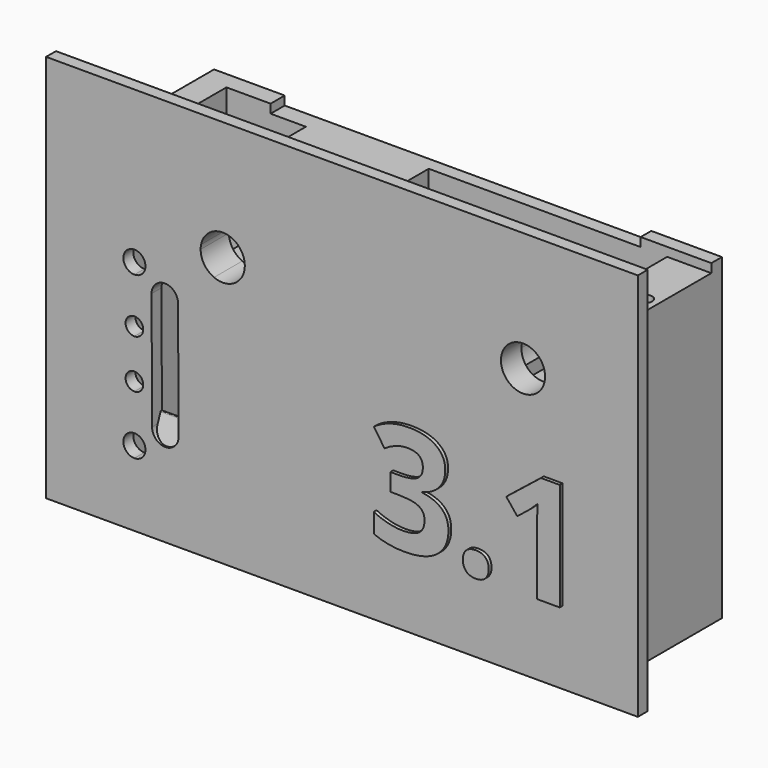
from build123d import *

# Parameters (mm, degrees)
F1_DEPTH      = 15
F2_W          = 15
F2_H          = 4
F3_DEPTH      = 25
F3_DEPTH_BACK = 1
F6_DEPTH      = 25
F7_DEPTH      = 15
F9_DEPTH      = 25
F10_W         = 27
F10_H         = 15
F11_DEPTH     = 2
F12_W         = 48
F12_H         = 36
F13_DEPTH     = 1.5
F14_W         = 48
F14_H         = 36
F15_DEPTH     = 1.5
F17_DEPTH     = 1.4
F18_W         = 8
F18_H         = 8.5
F19_DEPTH     = 11
F21_DEPTH     = 25
F22_W         = 16
F22_H         = 31
F23_DEPTH     = 2.5
F25_DEPTH     = 3.5
F26_W         = 2
F26_H         = 36
F27_DEPTH     = 3
F28_W         = 1.4
F28_H         = 44
F29_DEPTH     = 7
F30_W         = 18.8729918897
F30_H         = 36
F31_DEPTH     = 3
F32_W         = 12
F32_H         = 0.4
F33_DEPTH     = 27
F35_DEPTH     = 3
F36_TEXT_SIZE = 17.1089046893
F37_DEPTH     = 0.4
F39_W         = 4.7157869264
F39_H         = 15
F40_DEPTH     = 8
F41_DEPTH     = 25
F42_R         = 2.5
F43_DEPTH     = 8
F45_DEPTH     = 4
F47_DEPTH     = 6.5
F48_W         = 41.5
F48_H         = 1
F49_DEPTH     = 2
F50_W         = 2
F50_H         = 3.182195127
F51_DEPTH     = 4
F52_R         = 0.8
F53_DEPTH     = 40
F54_R         = 1.1997866049
F55_DEPTH     = 4


# Not quite as in the source:
# - Text() gives the source's letters only with a copy of the font that has no kerning and outlines rounded to 1/6400 em; it was checked with that copy


with BuildPart() as f1:
    # F0 (on Front) → F1 (new body)
    with BuildSketch(Plane.XZ):
        Polygon((6.5, 28.2073154487), (-6.5, 28.2073154487), (-6.5, 24.2073154487), (-24, -6.7926845513), (-22.5, -6.7926845513), (-5, 24.2073154487), (5, 24.2073154487), (22.5, -6.7926845513), (24, -6.7926845513), (6.5, 24.2073154487), align=None)
    extrude(amount=F1_DEPTH)

    # F2 (on face) → F3 (join, two sides)
    with BuildSketch(Plane(origin=(-6.5, 0, 0), x_dir=(0, -1, 0), z_dir=(-1, 0, 0))) as f3_sk:
        with Locations((7.5, 26.2073154487)):
            Rectangle(F2_W, F2_H)
    extrude(amount=-F3_DEPTH)
    extrude(f3_sk.sketch, amount=F3_DEPTH_BACK)

    # F4 (on face) → F6 (cut)
    with BuildSketch(Plane.XY.offset(28.2073154487)):
        with BuildLine():
            ThreePointArc((5.3, -7.5), (0, -2.2), (-5.3, -7.5))
            Line((-5.3, -7.5), (5.3, -7.5))
        make_face()
        with BuildLine():
            Line((5.3, -7.5), (-5.3, -7.5))
            ThreePointArc((-5.3, -7.5), (0, -12.8), (5.3, -7.5))
        make_face()
    extrude(amount=-F6_DEPTH, mode=Mode.SUBTRACT)

    # F5 (on face) → F7 (join)
    with BuildSketch(Plane(origin=(0, 0, 0), x_dir=(-1, 0, 0), z_dir=(0, 1, 0))):
        Polygon((22.5, -6.7926845513), (24, -6.7926845513), (24, 28.2073154487), (-24, 28.2073154487), (-24, -6.7926845513), (-22.5, -6.7926845513), (-5, 24.2073154487), (5, 24.2073154487), align=None)
    extrude(amount=-F7_DEPTH)

    # F8 (on face) → F9 (cut)
    with BuildSketch(Plane.XY.offset(28.2073154487)):
        with BuildLine():
            ThreePointArc((5.3, -7.5), (0, -2.2), (-5.3, -7.5))
            Line((-5.3, -7.5), (5.3, -7.5))
        make_face()
        with BuildLine():
            Line((5.3, -7.5), (-5.3, -7.5))
            ThreePointArc((-5.3, -7.5), (0, -12.8), (5.3, -7.5))
        make_face()
    extrude(amount=-F9_DEPTH, mode=Mode.SUBTRACT)

    # F10 (on face) → F11 (cut)
    with BuildSketch(Plane.XY.offset(28.2073154487)):
        with Locations((5.5, -7.5)):
            Rectangle(F10_W, F10_H)
    extrude(amount=-F11_DEPTH, mode=Mode.SUBTRACT)

    # F12 (on face) → F13 (join)
    with BuildSketch(Plane(origin=(0, 0, 0), x_dir=(-1, 0, 0), z_dir=(0, 1, 0))):
        with Locations((0, 11.2073154487)):
            Rectangle(F12_W, F12_H)
    extrude(amount=F13_DEPTH)

    # F14 (on face) → F15 (join)
    with BuildSketch(Plane.XZ.offset(15)):
        with Locations((0, 11.2073154487)):
            Rectangle(F14_W, F14_H)
    extrude(amount=F15_DEPTH)

    # F16 (on face) → F17 (join)
    with BuildSketch(Plane.XZ.offset(16.5)):
        Polygon((30, 37.2073154487), (-30, 37.2073154487), (-30, 29.2073154487), (-30, -6.7926845513), (30, -6.7926845513), (30, 29.2073154487), align=None)
    extrude(amount=F17_DEPTH)

    # F18 (on face) → F19 (cut)
    with BuildSketch(Plane(origin=(-24, 0, 0), x_dir=(0, -1, 0), z_dir=(-1, 0, 0))):
        with Locations((9.9, 24.4573154487)):
            Rectangle(F18_W, F18_H)
    extrude(amount=-F19_DEPTH, mode=Mode.SUBTRACT)

    # F20 (on face) → F21 (cut)
    with BuildSketch(Plane(origin=(0, -13.9, 0), x_dir=(-1, 0, 0), z_dir=(0, 1, 0))):
        with BuildLine():
            ThreePointArc((19.5, 23.7073154487), (19.4873403825, 23.9585878537), (19.4494897428, 24.2073154487))
            Line((19.4494897428, 24.2073154487), (16.7857142857, 24.2073154487))
            Line((16.7857142857, 24.2073154487), (17.9847982464, 21.4094528736))
            ThreePointArc((17.9847982464, 21.4094528736), (19.0871027306, 22.3310879268), (19.5, 23.7073154487))
        make_face()
        with BuildLine():
            Line((16.7857142857, 24.2073154487), (19.4494897428, 24.2073154487))
            ThreePointArc((19.4494897428, 24.2073154487), (18.1594859872, 25.9221726101), (16.0152017536, 26.0051780237))
            Line((16.0152017536, 26.0051780237), (16.7857142857, 24.2073154487))
        make_face()
        with BuildLine():
            Line((17.9847982464, 21.4094528736), (16.7857142857, 24.2073154487))
            Line((16.7857142857, 24.2073154487), (14.5505102572, 24.2073154487))
            ThreePointArc((14.5505102572, 24.2073154487), (15.4209689547, 21.7691046867), (17.9847982464, 21.4094528736))
        make_face()
        with BuildLine():
            Line((14.5505102572, 24.2073154487), (16.7857142857, 24.2073154487))
            Line((16.7857142857, 24.2073154487), (16.0152017536, 26.0051780237))
            ThreePointArc((16.0152017536, 26.0051780237), (15.061789238, 25.286346494), (14.5505102572, 24.2073154487))
        make_face()
    extrude(amount=-F21_DEPTH, mode=Mode.SUBTRACT)

    # F22 (on face) → F23 (cut)
    with BuildSketch(Plane(origin=(-24, 0, 0), x_dir=(0, -1, 0), z_dir=(-1, 0, 0))):
        with Locations((8.5, 13.7073154487)):
            Rectangle(F22_W, F22_H)
    extrude(amount=-F23_DEPTH, mode=Mode.SUBTRACT)

    # F24 (on face) → F25 (join)
    with BuildSketch(Plane(origin=(-24, 0, 0), x_dir=(0, -1, 0), z_dir=(-1, 0, 0))):
        Polygon((0.5, 29.2073154487), (-1.5, 29.2073154487), (-1.5, -6.7926845513), (16.5, -6.7926845513), (16.5, -1.7926845513), (0.5, -1.7926845513), (0.5, 28.2073154487), align=None)
    extrude(amount=F25_DEPTH)

    # F26 (on face) → F27 (join)
    with BuildSketch(Plane(origin=(-27.5, 0, 0), x_dir=(0, -1, 0), z_dir=(-1, 0, 0))):
        with Locations((-0.5, 11.2073154487)):
            Rectangle(F26_W, F26_H)
    extrude(amount=F27_DEPTH)

    # F28 (on face) → F29 (join)
    with BuildSketch(Plane(origin=(-30, 0, 0), x_dir=(0, -1, 0), z_dir=(-1, 0, 0))):
        with Locations((17.2, 15.2073154487)):
            Rectangle(F28_W, F28_H)
    extrude(amount=F29_DEPTH)

    # F30 (on face) → F31 (join)
    with BuildSketch(Plane(origin=(-30.5, 0, 0), x_dir=(0, -1, 0), z_dir=(-1, 0, 0))):
        with Locations((7.9364959449, 11.2073154487)):
            Rectangle(F30_W, F30_H)
    extrude(amount=F31_DEPTH)

    # F32 (on face) → F33 (cut)
    with BuildSketch(Plane.XY.offset(29.2073154487)):
        with Locations((-26, -16.3)):
            Rectangle(F32_W, F32_H)
    extrude(amount=-F33_DEPTH, mode=Mode.SUBTRACT)

    # F34 (on face) → F35 (cut)
    with BuildSketch(Plane.XZ.offset(17.9)):
        with BuildLine():
            ThreePointArc((-25.75, 20.0012622166), (-26.1161165235, 20.8851456931), (-27, 21.2512622166))
            Line((-27, 21.2512622166), (-27, 18.7512622166))
            ThreePointArc((-27, 18.7512622166), (-26.1161165235, 19.1173787402), (-25.75, 20.0012622166))
        make_face()
        with BuildLine():
            ThreePointArc((-25.75, 1.7012622166), (-26.1161165235, 2.5851456931), (-27, 2.9512622166))
            Line((-27, 2.9512622166), (-27, 0.4512622166))
            ThreePointArc((-27, 0.4512622166), (-26.1161165235, 0.8173787402), (-25.75, 1.7012622166))
        make_face()
        with BuildLine():
            Line((-27, 0.4512622166), (-27, 2.9512622166))
            ThreePointArc((-27, 2.9512622166), (-28.25, 1.7012622166), (-27, 0.4512622166))
        make_face()
        with BuildLine():
            ThreePointArc((-26, 8.1012622166), (-26.2928932188, 8.8083689978), (-27, 9.1012622166))
            Line((-27, 9.1012622166), (-27, 7.1012622166))
            ThreePointArc((-27, 7.1012622166), (-26.2928932188, 7.3941554355), (-26, 8.1012622166))
        make_face()
        with BuildLine():
            Line((-27, 7.1012622166), (-27, 9.1012622166))
            ThreePointArc((-27, 9.1012622166), (-28, 8.1012622166), (-27, 7.1012622166))
        make_face()
        with BuildLine():
            ThreePointArc((-26, 13.6012622166), (-26.2928932188, 14.3083689978), (-27, 14.6012622166))
            Line((-27, 14.6012622166), (-27, 12.6012622166))
            ThreePointArc((-27, 12.6012622166), (-26.2928932188, 12.8941554355), (-26, 13.6012622166))
        make_face()
        with BuildLine():
            Line((-27, 12.6012622166), (-27, 14.6012622166))
            ThreePointArc((-27, 14.6012622166), (-28, 13.6012622166), (-27, 12.6012622166))
        make_face()
        with BuildLine():
            Line((-27, 18.7512622166), (-27, 21.2512622166))
            ThreePointArc((-27, 21.2512622166), (-28.25, 20.0012622166), (-27, 18.7512622166))
        make_face()
        with BuildLine():
            Line((-25.0565237088, 17.488491505), (-25, 4.2106055044))
            ThreePointArc((-25, 4.2106055044), (-23.499203428, 2.7012624439), (-22.0000693935, 4.212256809))
            Line((-22.0000693935, 4.212256809), (-22.0565780734, 17.5012622166))
            ThreePointArc((-22.0565780734, 17.5012622166), (-23.5565780734, 19.0012622166), (-25.0565780734, 17.5012622166))
            ThreePointArc((-25.0565780734, 17.5012622166), (-25.0565644822, 17.494876803), (-25.0565237088, 17.488491505))
        make_face()
    extrude(amount=-F35_DEPTH, mode=Mode.SUBTRACT)

    # F36 (on face) → F37 (join)
    with BuildSketch(Plane.XZ.offset(17.9)):
        with Locations((-0.2313149162, 1.5029550996)):
            Text('3.1', F36_TEXT_SIZE, font='Open Sans', font_style=FontStyle.BOLD, text_align=(TextAlign.LEFT, TextAlign.BOTTOM))
    extrude(amount=F37_DEPTH)

    # F39 (on face) → F40 (cut)
    with BuildSketch(Plane.XY.offset(28.2073154487)):
        with Locations((16.6421065368, -7.5)):
            Rectangle(F39_W, F39_H)
    extrude(amount=-F40_DEPTH, mode=Mode.SUBTRACT)

    # F38 (on face) → F41 (join)
    with BuildSketch(Plane(origin=(-24.9816228181, 0, -0.1063462943), x_dir=(0, 1, 0), z_dir=(0.9999909392, 0, 0.0042569425))):
        with BuildLine():
            Line((-16.6931281305, 5.3539588312), (-17.9, 2.3169909142))
            Line((-17.9, 2.3169909142), (-16.5, 2.3169909142))
            Line((-16.5, 2.3169909142), (-16.5, 5.3169909142))
            Line((-16.5, 5.3169909142), (-16.5, 5.4136584855))
            Line((-16.5, 5.4136584855), (-16.5966086841, 5.4170321351))
            ThreePointArc((-16.5966086841, 5.4170321351), (-16.6548614343, 5.4007875541), (-16.6931281305, 5.3539588312))
        make_face()
    extrude(amount=F41_DEPTH)

    # F42 (on face) → F43 (cut)
    with BuildSketch(Plane.XZ.offset(17.9)):
        with Locations((17, 23.7073154487)):
            Circle(F42_R)
    extrude(amount=-F43_DEPTH, mode=Mode.SUBTRACT)

    # F44 (on face) → F45 (cut)
    with BuildSketch(Plane(origin=(0, -15, 0), x_dir=(-1, 0, 0), z_dir=(0, 1, 0))):
        with BuildLine():
            ThreePointArc((-19.834218055, 23.2073154487), (-16.834218055, 20.2073154487), (-13.834218055, 23.2073154487))
            ThreePointArc((-13.834218055, 23.2073154487), (-16.5833392742, 26.196807017), (-19.7922579466, 23.7073154487))
            ThreePointArc((-19.7922579466, 23.7073154487), (-19.8237096234, 23.4581942295), (-19.834218055, 23.2073154487))
        make_face()
    extrude(amount=F45_DEPTH, mode=Mode.SUBTRACT)

    # F46 (on face) → F47 (join)
    with BuildSketch(Plane.XY.offset(26.2073154487)):
        Polygon((13.3841438219, -7.5), (14.2842130736, -7.5), (20.0731083751, -7.5), (20.0731083751, 0.6800028495), (13.3841438219, 0.6800028495), align=None)
    extrude(amount=-F47_DEPTH)

    # F48 (on face) → F49 (cut)
    with BuildSketch(Plane(origin=(0, 1.5, 0), x_dir=(-1, 0, 0), z_dir=(0, 1, 0))):
        with Locations((4.75, 28.7073154487)):
            Rectangle(F48_W, F48_H)
    extrude(amount=-F49_DEPTH, mode=Mode.SUBTRACT)

    # F50 (on face) → F51 (cut)
    with BuildSketch(Plane.XY.offset(28.2073154487)):
        with Locations((20, -11.0088186339)):
            Rectangle(F50_W, F50_H)
    extrude(amount=-F51_DEPTH, mode=Mode.SUBTRACT)

    # F52 (on face) → F53 (cut)
    with BuildSketch(Plane(origin=(0, 0, -6.7926845513), x_dir=(1, 0, 0), z_dir=(0, 0, -1))):
        with Locations((22.5, 7.5)):
            Circle(F52_R)
    extrude(amount=-F53_DEPTH, mode=Mode.SUBTRACT)

    # F54 (on face) → F55 (cut)
    with BuildSketch(Plane(origin=(19, 0, 0), x_dir=(0, -1, 0), z_dir=(-1, 0, 0))):
        with Locations((8.7002133951, 21.4263591915)):
            Circle(F54_R)
    extrude(amount=-F55_DEPTH, mode=Mode.SUBTRACT)


solid = f1.part
